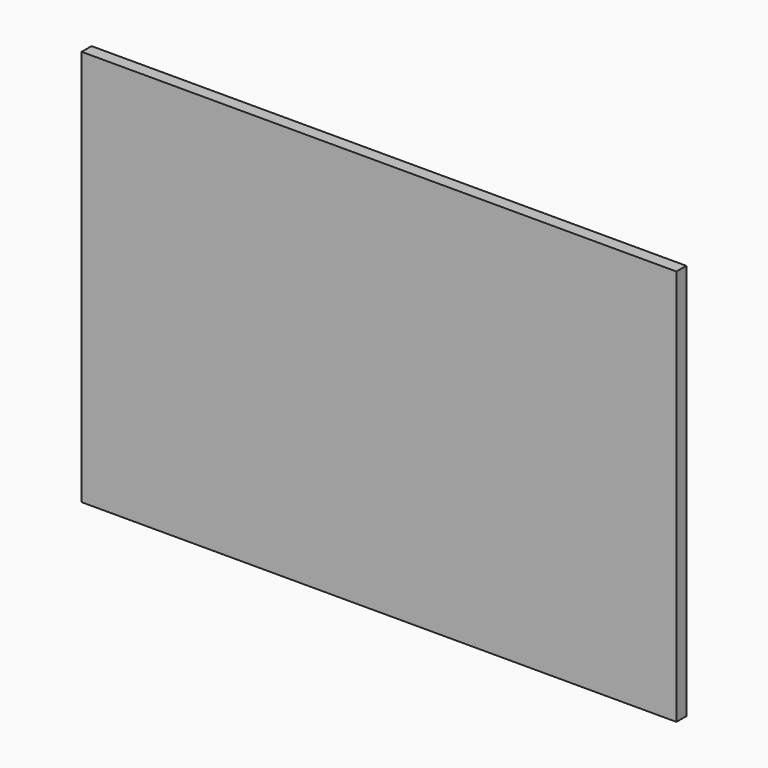
from build123d import *

# Parameters (mm, degrees)
F0_W     = 381
F0_H     = 254
F1_DEPTH = 7.9375


# Not quite as in the source:
# - a length typed as a fraction of an inch, garbled in the dataset ("3 / 203.2 mm" for 3/8 in), is restored


with BuildPart() as f1:
    # F0 (on Front) → F1 (new body)
    with BuildSketch(Plane.XZ):
        with Locations((128.397805352, 95.5933926851)):
            Rectangle(F0_W, F0_H)
    extrude(amount=F1_DEPTH)


solid = f1.part
